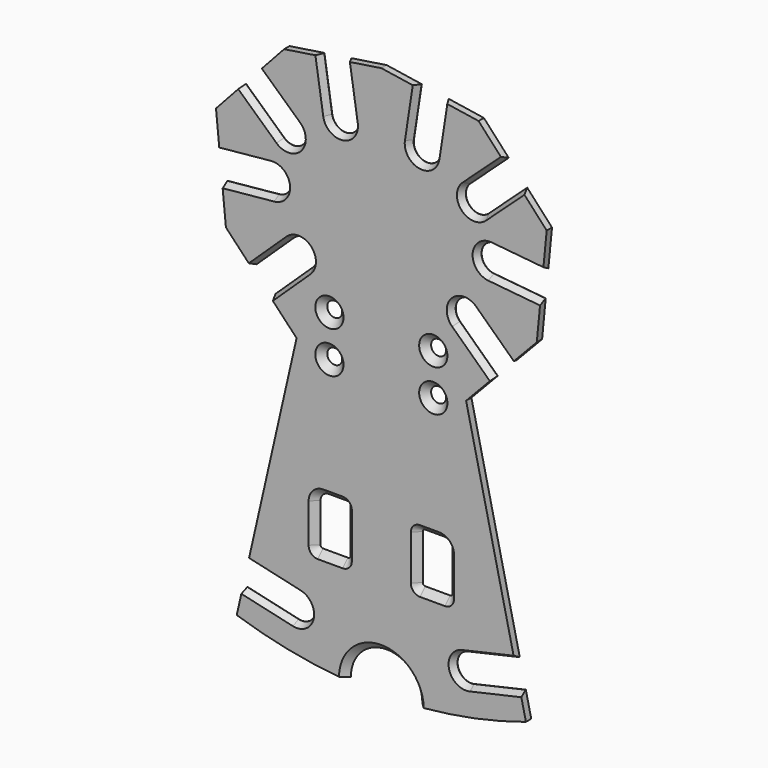
from build123d import *

# Parameters (mm, degrees)
F0_R     = 9
F1_DEPTH = 8
F2_R     = 3
F3_SIZE  = 7.99999
F4_SIZE2 = 7.7942286341
F4_SIZE  = 4.5


# Not quite as in the source:
# - a fillet or chamfer is up to 0.001 mm smaller than in the source, because OpenCascade refuses the exact size
# - ends of sketch curves that miss each other by under 0.0002 mm in the source are joined


with BuildPart() as f1:
    # F0 (on Front) → F1 (new body)
    with BuildSketch(Plane.XZ):
        with BuildLine():
            ThreePointArc((-43, -330.994167), (0, -287.994167), (43, -330.994167))
            ThreePointArc((43, -330.994167), (109.276026714, -321.904147751), (174.0000001055, -304.9941673237))
            Line((174.0000001055, -304.9941673237), (167.462801, -276.227606))
            Line((167.462801, -276.227606), (105.54156, -290.299203))
            ThreePointArc((105.54156, -290.299203), (85.7953886494, -277.8658315797), (98.2287608958, -258.1196605414))
            Line((98.2287608958, -258.1196605414), (160.150002, -244.048063))
            Line((160.150002, -244.048063), (101.992538, 11.87045))
            Line((101.992538, 11.87045), (133.663965, 45.228522))
            Line((133.663965, 45.228522), (88.338787, 88.261977))
            ThreePointArc((88.338787, 88.261977), (87.7337722092, 111.5886563014), (111.0604515643, 112.1936705411))
            Line((111.0604515643, 112.1936705411), (156.385629, 69.160216))
            Line((156.385629, 69.160216), (187.038105, 101.445071))
            Line((187.038105, 101.445071), (191.402576, 146.180902))
            Line((191.402576, 146.180902), (129.197911, 152.24965))
            ThreePointArc((129.197911, 152.24965), (114.3780295485, 170.2738304953), (132.4022099517, 185.0937125046))
            Line((132.4022099517, 185.0937125046), (194.606875, 179.024965))
            Line((194.606875, 179.024965), (198.96141, 223.658948))
            Line((198.96141, 223.658948), (169.162302, 256.167065))
            Line((169.162302, 256.167065), (123.090168, 213.934276))
            ThreePointArc((123.090168, 213.934276), (99.7776684169, 214.9478629238), (100.7912561729, 238.2603628114))
            Line((100.7912561729, 238.2603628114), (146.863389, 280.493152))
            Line((146.863389, 280.493152), (117.000674, 313.07066))
            Line((117.000674, 313.07066), (74.908309, 319.518852))
            Line((74.908309, 319.518852), (65.444247, 257.739555))
            ThreePointArc((65.444247, 257.739555), (46.6359995191, 243.928333625), (32.8247775616, 262.7365800672))
            Line((32.8247775616, 262.7365800672), (42.288841, 324.515877))
            Line((42.288841, 324.515877), (0, 330.994168))
            Line((0, 330.994168), (-42.288841, 324.515877))
            Line((-42.288841, 324.515877), (-32.824778, 262.73658))
            ThreePointArc((-32.824778, 262.73658), (-46.6360005191, 243.928333625), (-65.4442472887, 257.7395549558))
            Line((-65.4442472887, 257.7395549558), (-74.908309, 319.518852))
            Line((-74.908309, 319.518852), (-117.000674, 313.07066))
            Line((-117.000674, 313.07066), (-146.86339, 280.493152))
            Line((-146.86339, 280.493152), (-100.791256, 238.260363))
            ThreePointArc((-100.791256, 238.260363), (-99.7776686659, 214.9478626521), (-123.0901688686, 213.9342761433))
            Line((-123.0901688686, 213.9342761433), (-169.162302, 256.167065))
            Line((-169.162302, 256.167065), (-198.96141, 223.658948))
            Line((-198.96141, 223.658948), (-194.606875, 179.024965))
            Line((-194.606875, 179.024965), (-132.40221, 185.093713))
            ThreePointArc((-132.40221, 185.093713), (-114.3780295485, 170.2738304953), (-129.1979109611, 152.2496496015))
            Line((-129.1979109611, 152.2496496015), (-191.402576, 146.180902))
            Line((-191.402576, 146.180902), (-187.038105, 101.445071))
            Line((-187.038105, 101.445071), (-156.385629, 69.160216))
            Line((-156.385629, 69.160216), (-111.060452, 112.193671))
            ThreePointArc((-111.060452, 112.193671), (-87.7337732092, 111.5886563014), (-88.3387874357, 88.2619774589))
            Line((-88.3387874357, 88.2619774589), (-133.663965, 45.228522))
            Line((-133.663965, 45.228522), (-101.992538, 11.87045))
            Line((-101.992538, 11.87045), (-160.150002, -244.048063))
            Line((-160.150002, -244.048063), (-98.228761, -258.119661))
            ThreePointArc((-98.228761, -258.119661), (-85.7953886494, -277.8658315797), (-105.5415600551, -290.2992032425))
            Line((-105.5415600551, -290.2992032425), (-167.462801, -276.227606))
            Line((-167.462801, -276.227606), (-174, -304.994167))
            ThreePointArc((-174, -304.994167), (-109.276026714, -321.904147751), (-43, -330.994167))
        make_face()
        with BuildLine():
            Line((-69.5, -145.994167), (-43.5, -145.994167))
            Line((-43.5, -145.994167), (-43.5, -205.994167))
            Line((-43.5, -205.994167), (-79.5, -205.994167))
            Line((-79.5, -205.994167), (-79.5, -155.994167))
            ThreePointArc((-79.5, -155.994167), (-76.5710678119, -148.9230991881), (-69.5, -145.994167))
        make_face(mode=Mode.SUBTRACT)
        with BuildLine():
            Line((43.5, -205.994167), (43.5, -145.994167))
            Line((43.5, -145.994167), (69.5, -145.994167))
            ThreePointArc((69.5, -145.994167), (76.5710678119, -148.9230991881), (79.5, -155.994167))
            Line((79.5, -155.994167), (79.5, -205.994167))
            Line((79.5, -205.994167), (43.5, -205.994167))
        make_face(mode=Mode.SUBTRACT)
        with Locations((-62.5, 2.005833)):
            Circle(F0_R, mode=Mode.SUBTRACT)
        with Locations((-62.5, 52.005833)):
            Circle(F0_R, mode=Mode.SUBTRACT)
        with Locations((62.5, 2.005833)):
            Circle(F0_R, mode=Mode.SUBTRACT)
        with Locations((62.5, 52.005833)):
            Circle(F0_R, mode=Mode.SUBTRACT)
    extrude(amount=F1_DEPTH)

    # F2
    f2_edges = [f1.edges().sort_by_distance(p)[0] for p in [
        (-43.5, -4, -205.994167),
        (79.5, -4, -205.994167),
        (43.5, -4, -205.994167),
        (-79.5, -4, -205.994167),
        (-43.5, -4, -145.994167),
        (43.5, -4, -145.994167),
    ]]
    fillet(f2_edges, radius=F2_R)

    # F3 (size 8 in the source; OpenCascade refuses exactly that, so slightly less here)
    f3_edges = [f1.edges().sort_by_distance(p)[0] for p in [
        (-71.5, -8, 52.005833),
        (53.5, -8, 52.005833),
        (-71.5, -8, 2.005833),
        (53.5, -8, 2.005833),
        (-58, -8, -145.994167),
        (58, -8, -145.994167),
        (0, -8, -287.994167),
    ]]
    chamfer(f3_edges, length=F3_SIZE)

    # F4
    f4_edges = [f1.edges().sort_by_distance(p)[0] for p in [
        (-133.72304, -8, 90.676943),
        (-163.504543, -8, 182.059339),
        (-123.827323, -8, 259.376757),
        (-37.556809, -8, 293.626229),
        (70.176278, -8, 288.629204),
        (123.827323, -8, 259.376757),
        (163.504542, -8, 182.059339),
        (133.72304, -8, 90.676943),
        (129.189381, -8, -251.083862),
        (-129.189381, -8, -251.083862),
    ]]
    f4_side = f1.faces().sort_by_distance((0, -8, 8.818439))[0]
    chamfer(f4_edges, length=F4_SIZE, length2=F4_SIZE2, reference=f4_side)


solid = f1.part
